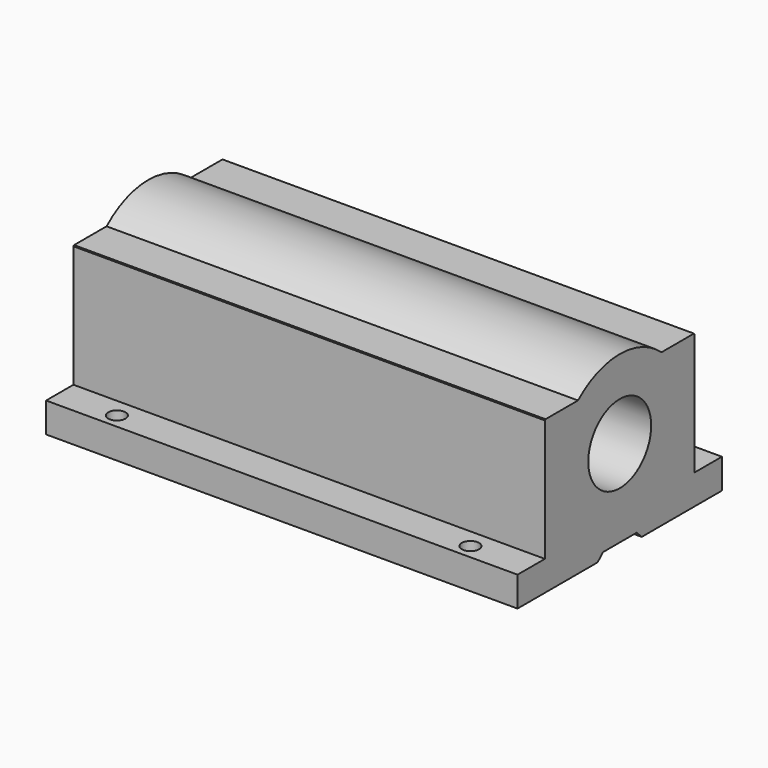
from build123d import *

# Parameters (mm, degrees)
F0_R     = 12.7063531766
F1_DEPTH = 76.2
F2_R     = 2.794
F3_DEPTH = 9.6578284142


# Not quite as in the source:
# - ends of sketch curves that miss each other by under 0.0002 mm in the source are joined


with BuildPart() as f1:
    # F0 (on Right) → F1 (new body, symmetric)
    with BuildSketch(Plane.YZ):
        with BuildLine():
            Line((-41.2956478239, -26.3029134567), (-8.8944472236, -26.3029134567))
            Line((-8.8944472236, -26.3029134567), (-6.8614307154, -24.2698969485))
            Line((-6.8614307154, -24.2698969485), (6.8614307154, -24.2698969485))
            Line((6.8614307154, -24.2698969485), (8.8944472236, -26.3029134567))
            Line((8.8944472236, -26.3029134567), (41.2956478239, -26.3029134567))
            Line((41.2956478239, -26.3029134567), (41.2956478239, -16.6460850425))
            Line((41.2956478239, -16.6460850425), (30.2411205603, -16.6460850425))
            Line((30.2411205603, -16.6460850425), (30.2411205603, 22.7436098049))
            Line((30.2411205603, 22.7436098049), (29.9869934967, 22.9977368684))
            Line((29.9869934967, 22.9977368684), (16.8568834417, 22.9977368684))
            ThreePointArc((16.8568834417, 22.9977368684), (0, 29.3509134567), (-16.8568829775, 22.9977363401))
            Line((-16.8568829775, 22.9977363401), (-29.9869934967, 22.9977368684))
            Line((-29.9869934967, 22.9977368684), (-30.2411205603, 22.7436098049))
            Line((-30.2411205603, 22.7436098049), (-30.2411205603, -16.6460850425))
            Line((-30.2411205603, -16.6460850425), (-41.2956478239, -16.6460850425))
            Line((-41.2956478239, -16.6460850425), (-41.2956478239, -26.3029134567))
        make_face()
        with Locations((0, 3.8619689845)):
            Circle(F0_R, mode=Mode.SUBTRACT)
    extrude(amount=F1_DEPTH, both=True)

    # F2 (on face) → F3 (cut, through all)
    with BuildSketch(Plane.XY.offset(-16.6460850425)):
        with Locations((57.15, 36.5125)):
            Circle(F2_R)
        with Locations((-57.15, 36.5125)):
            Circle(F2_R)
        with Locations((-57.15, -36.5125)):
            Circle(F2_R)
        with Locations((57.15, -36.5125)):
            Circle(F2_R)
    extrude(amount=-F3_DEPTH, mode=Mode.SUBTRACT)


solid = f1.part
